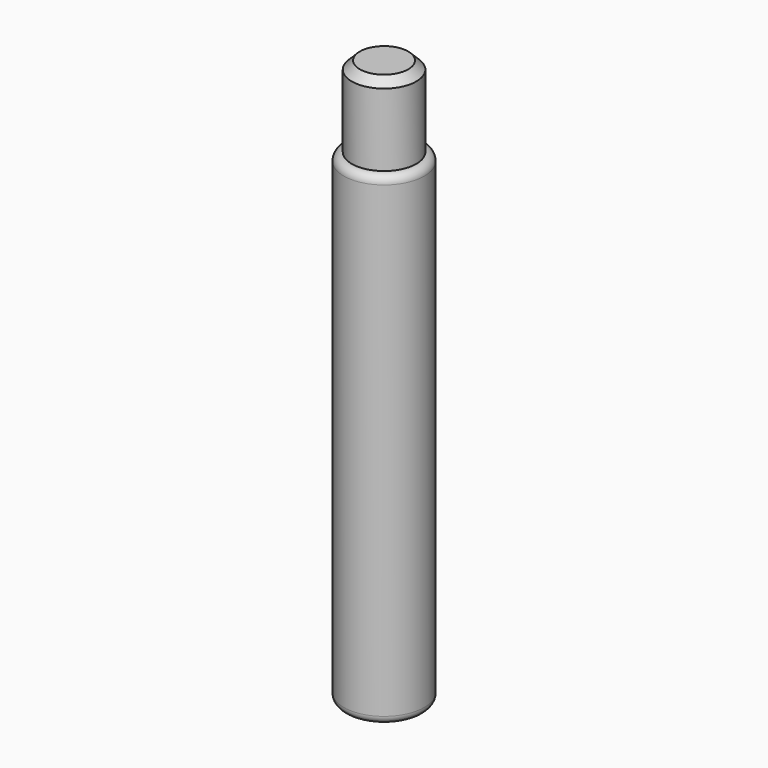
from build123d import *

# Parameters (mm, degrees)
F0_R     = 5
F1_DEPTH = 50
F2_R     = 1
F3_DEPTH = 10
F4_R     = 1
F5_R     = 4
F6_DEPTH = 10
F7_SIZE  = 1
F8_DEPTH = 25


with BuildPart() as f1:
    # F0 (on Top) → F1 (new body)
    with BuildSketch(Plane.XY):
        Circle(F0_R)
    extrude(amount=F1_DEPTH)

    # F2
    f2_edges = [f1.edges().sort_by_distance(p)[0] for p in [
        (-5, 0, 0),
    ]]
    fillet(f2_edges, radius=F2_R)

    # F3 (add): a face of the model
    f3_faces = [f1.faces().sort_by_distance(p)[0] for p in [
        (0, 0, 50),
    ]]
    extrude(f3_faces, amount=F3_DEPTH)

    # F4
    f4_edges = [f1.edges().sort_by_distance(p)[0] for p in [
        (-5, 0, 60),
    ]]
    fillet(f4_edges, radius=F4_R)


with BuildPart() as f6:
    # F5 (on face) → F6 (new body)
    with BuildSketch(Plane.XY.offset(60)):
        Circle(F5_R)
    extrude(amount=F6_DEPTH)

    # F7
    f7_edges = [f6.edges().sort_by_distance(p)[0] for p in [
        (-4, 0, 70),
    ]]
    chamfer(f7_edges, length=F7_SIZE)


with BuildPart() as f8:
    # F8 (new): a face of the model
    f8_faces = [f6.part.faces().sort_by_distance(p)[0] for p in [
        (0, 0, 70),
    ]]
    extrude(f8_faces, amount=-F8_DEPTH)


solid = Compound([f1.part, f6.part, f8.part])
